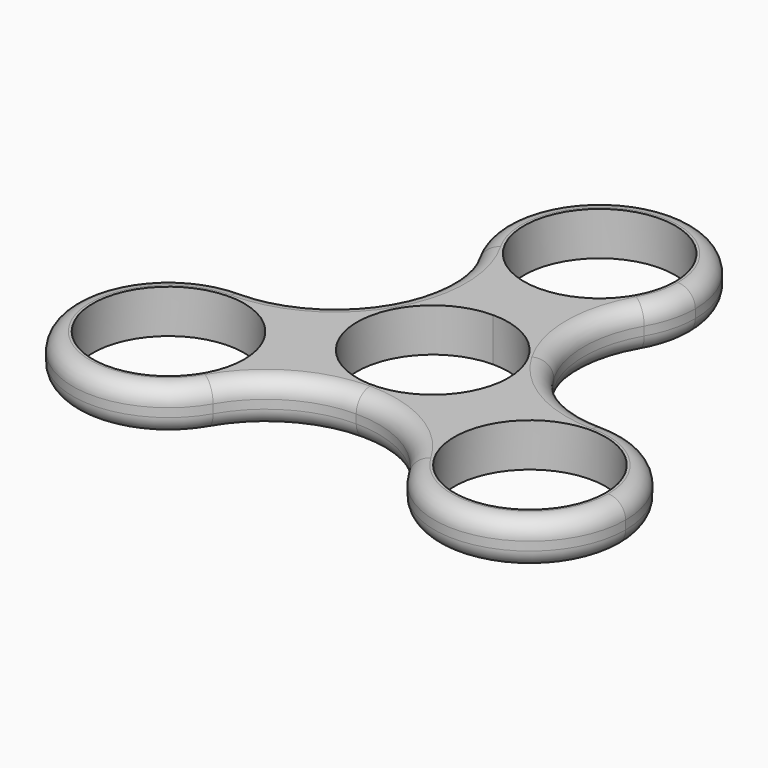
from build123d import *

# Parameters (mm, degrees)
F0_R     = 11.049
F1_DEPTH = 6.35
F2_R     = 2.54


with BuildPart() as f1:
    # F0 (on Top) → F1 (new body)
    with BuildSketch(Plane.XY):
        with BuildLine():
            ThreePointArc((0, 11.049), (7.8128228253, 7.8128228253), (11.049, 0))
            ThreePointArc((11.049, 0), (-2.8596916293, -10.6725144547), (-9.5687146864, 5.5245))
            Line((-9.5687146864, 5.5245), (-12.0983748909, 6.985))
            ThreePointArc((-12.0983748842, 6.9850000115), (-12.0983748972, -6.9849999891), (-1.19e-08, -13.97))
            ThreePointArc((-1.19e-08, -13.97), (9.878281729, -9.8782817374), (13.97, 0))
            ThreePointArc((13.97, 0), (13.4939838051, 3.615702016), (12.0983749365, 6.984999921))
            ThreePointArc((12.0983749365, 6.984999921), (6.9850000395, 12.0983748681), (0, 13.97))
            Line((0, 13.97), (0, 11.049))
        make_face()
        with BuildLine():
            ThreePointArc((-9.5687146864, 5.5245), (-5.5245, 9.5687146864), (0, 11.049))
            Line((0, 11.049), (0, 13.97))
            ThreePointArc((0, 13.97), (-6.9849999943, 12.0983748942), (-12.0983748842, 6.9850000115))
            Line((-12.0983748909, 6.985), (-9.5687146864, 5.5245))
        make_face()
        with BuildLine():
            Line((0, 16.51), (0, 13.97))
            ThreePointArc((0, 13.97), (6.9850000395, 12.0983748681), (12.0983749365, 6.984999921))
            ThreePointArc((12.0983749365, 6.984999921), (9.8864543073, 15.2399999544), (12.0983748909, 23.495))
            ThreePointArc((12.0983748909, 23.495), (6.985, 18.3816251091), (0, 16.51))
        make_face()
        with BuildLine():
            ThreePointArc((-12.0983748842, 6.9850000115), (-6.9849999943, 12.0983748942), (0, 13.97))
            Line((0, 13.97), (0, 16.51))
            ThreePointArc((0, 16.51), (-6.985, 18.3816251091), (-12.0983748909, 23.495))
            ThreePointArc((-12.0983748909, 23.495), (-9.8864543073, 15.2400000066), (-12.0983748842, 6.9850000115))
        make_face()
        with BuildLine():
            ThreePointArc((-1.19e-08, -13.97), (-12.0983748972, -6.9849999891), (-12.0983748842, 6.9850000115))
            ThreePointArc((-12.0983748842, 6.9850000115), (-18.1414543016, 0.9419205868), (-26.3964543073, -1.27))
            ThreePointArc((-26.3964543073, -1.27), (-16.5181725742, -5.3617182668), (-12.4264543073, -15.24))
            ThreePointArc((-12.4264543073, -15.24), (-12.9024705141, -18.8557020601), (-14.2980794165, -22.225))
            ThreePointArc((-14.2980794165, -22.225), (-8.2550000052, -16.1819205865), (-1.19e-08, -13.97))
        make_face()
        with BuildLine():
            ThreePointArc((26.3964543073, -1.27), (18.1414543468, 0.9419205607), (12.0983749365, 6.984999921))
            ThreePointArc((12.0983749365, 6.984999921), (13.4939838051, 3.615702016), (13.97, 0))
            ThreePointArc((13.97, 0), (9.878281729, -9.8782817374), (-1.19e-08, -13.97))
            ThreePointArc((-1.19e-08, -13.97), (8.2549999948, -16.1819205805), (14.2980794165, -22.225))
            ThreePointArc((14.2980794165, -22.225), (14.2980794165, -8.255), (26.3964543073, -1.27))
        make_face()
        with BuildLine():
            ThreePointArc((-12.0983748909, 23.495), (-6.985, 18.3816251091), (0, 16.51))
            ThreePointArc((0, 16.51), (6.985, 18.3816251091), (12.0983748909, 23.495))
            ThreePointArc((12.0983748909, 23.495), (13.4939837933, 26.8642979399), (13.97, 30.48))
            ThreePointArc((13.97, 30.48), (-3.6157020601, 43.9739837933), (-12.0983748909, 23.495))
        make_face()
        with BuildLine():
            ThreePointArc((11.049, 30.48), (7.8128228253, 22.6671771747), (0, 19.431))
            ThreePointArc((0, 19.431), (-7.8128228253, 38.2928228253), (11.049, 30.48))
        make_face(mode=Mode.SUBTRACT)
        with BuildLine():
            ThreePointArc((-12.4264543073, -15.24), (-16.5181725742, -5.3617182668), (-26.3964543073, -1.27))
            ThreePointArc((-26.3964543073, -1.27), (-38.4948291982, -22.225), (-14.2980794165, -22.225))
            ThreePointArc((-14.2980794165, -22.225), (-12.9024705141, -18.8557020601), (-12.4264543073, -15.24))
        make_face()
        with Locations((-26.3964543073, -15.24)):
            Circle(F0_R, mode=Mode.SUBTRACT)
        with BuildLine():
            ThreePointArc((40.3664543073, -15.24), (36.2747360405, -5.3617182668), (26.3964543073, -1.27))
            ThreePointArc((26.3964543073, -1.27), (14.2980794165, -8.255), (14.2980794165, -22.225))
            ThreePointArc((14.2980794165, -22.225), (30.0121563674, -28.7339837933), (40.3664543073, -15.24))
        make_face()
        with Locations((26.3964543073, -15.24)):
            Circle(F0_R, mode=Mode.SUBTRACT)
    extrude(amount=F1_DEPTH)

    # F2
    f2_edges = [f1.edges().sort_by_distance(p)[0] for p in [
        (0, -13.97, 6.35),
        (0, -13.97, 0),
        (-12.098375, 6.985, 0),
        (-12.098375, 6.985, 6.35),
        (-38.494829, -22.225, 0),
        (-38.494829, -22.225, 6.35),
        (38.494829, -22.225, 0),
        (38.494829, -22.225, 6.35),
        (12.098375, 6.985, 0),
        (12.098375, 6.985, 6.35),
        (0, 44.45, 0),
        (0, 44.45, 6.35),
    ]]
    fillet(f2_edges, radius=F2_R)


solid = f1.part
